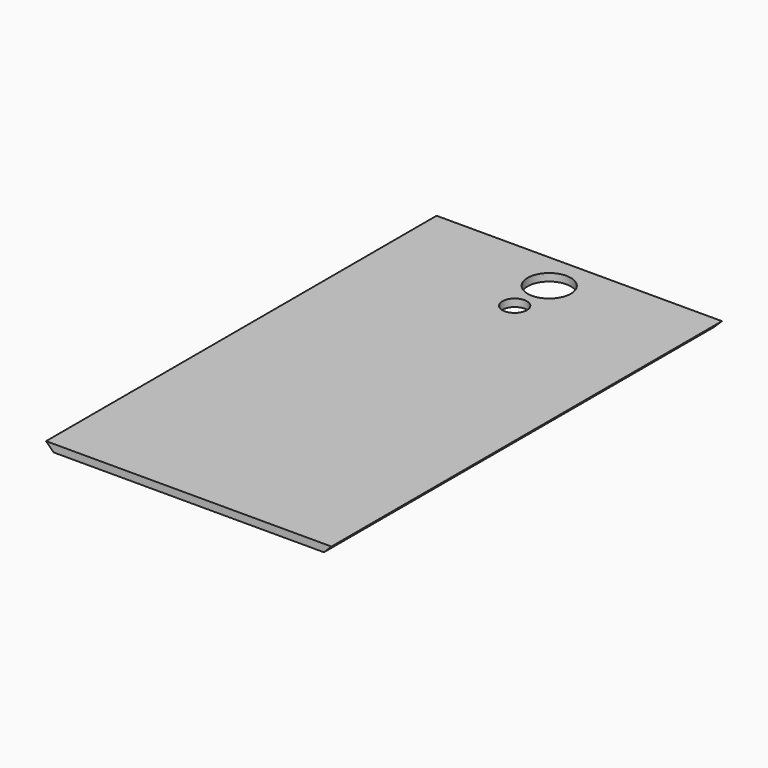
from build123d import *

# Parameters (mm, degrees)
F0_W     = 96.52
F0_H     = 165.1
F0_R     = 4.1275
F0_R_2   = 7.3025
F1_DEPTH = 2.54
F2_SIZE  = 2.53999


# Not quite as in the source:
# - a fillet or chamfer is up to 0.001 mm smaller than in the source, because OpenCascade refuses the exact size


with BuildPart() as f1:
    # F0 (on Top) → F1 (new body)
    with BuildSketch(Plane.XY):
        Rectangle(F0_W, F0_H)
        with Locations((0, 55.245)):
            Circle(F0_R, mode=Mode.SUBTRACT)
        with Locations((0, 69.85)):
            Circle(F0_R_2, mode=Mode.SUBTRACT)
    extrude(amount=F1_DEPTH)

    # F2 (size 2.54 in the source; OpenCascade refuses exactly that, so slightly less here)
    f2_edges = [f1.edges().sort_by_distance(p)[0] for p in [
        (-48.26, 0, 0),
        (48.26, 0, 0),
    ]]
    chamfer(f2_edges, length=F2_SIZE)


solid = f1.part
